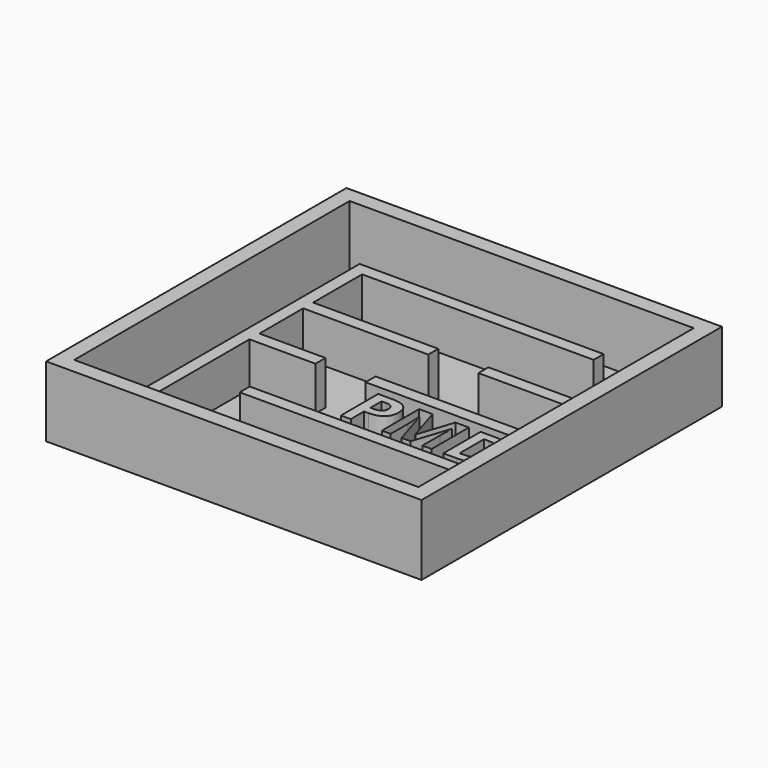
from build123d import *

# Parameters (mm, degrees)
F0_W         = 38.1
F0_H         = 38.1
F1_DEPTH     = 0.79375
F2_W         = 38.1
F2_H         = 38.1
F2_W_2       = 34.925
F2_H_2       = 34.925
F3_DEPTH     = 6.35
F4_R         = 1.27
F5_DEPTH     = 0.396875
F4_W         = 10.795
F4_H         = 1.27
F4_W_2       = 16.7933495293
F4_W_3       = 23.495
F4_W_4       = 12.2181028306
F4_W_5       = 11.1757950872
F6_DEPTH     = 4.445
F4_TEXT_SIZE = 6.6178126468
F7_DEPTH     = 4.445


# Not quite as in the source:
# - Text() gives the source's letters only with a copy of the font that has no kerning and outlines rounded to 1/6400 em; it was checked with that copy


with BuildPart() as f1:
    # F0 (on Top) → F1 (new body)
    with BuildSketch(Plane.XY):
        with Locations((7.1995537728, -11.629379993)):
            Rectangle(F0_W, F0_H)
    extrude(amount=F1_DEPTH)

    # F2 (on face) → F3 (join)
    with BuildSketch(Plane.XY.offset(0.79375)):
        with Locations((7.1995537728, -11.629379993)):
            Rectangle(F2_W, F2_H)
        with Locations((7.1995537728, -11.629379993)):
            Rectangle(F2_W_2, F2_H_2, mode=Mode.SUBTRACT)
    extrude(amount=F3_DEPTH)

    # F4 (on face) → F5 (cut)
    with BuildSketch(Plane.XY.offset(0.79375)):
        with Locations((-7.7175865881, -26.8155727535)):
            Circle(F4_R)
        with Locations((21.5233564377, -24.9188905582)):
            Circle(F4_R)
    extrude(amount=-F5_DEPTH, mode=Mode.SUBTRACT)

    # F4 (on face) → F6 (join)
    with BuildSketch(Plane.XY.offset(0.79375)):
        Polygon((-5.1829462272, 0.753120007), (-5.1829462272, -29.091879993), (-3.9129462272, -29.091879993), (-3.9129462272, -28.7239273232), (-3.9129462272, -27.4539273232), (-3.9129462272, -14.804379993), (2.7887042435, -14.804379993), (2.7887042435, -13.534379993), (-3.9129462272, -13.534379993), (-3.9129462272, -7.992786257), (8.7870537728, -7.992786257), (8.7870537728, -6.722786257), (-3.9129462272, -6.722786257), (-3.9129462272, -0.516879993), (19.5820537728, -0.516879993), (19.5820537728, 0.753120007), align=None)
        with Locations((19.2645537728, -7.357786257)):
            Rectangle(F4_W, F4_H)
        with Locations((16.2653790082, -14.169379993)):
            Rectangle(F4_W_2, F4_H)
        with Locations((12.9145537728, -21.7488537931)):
            Rectangle(F4_W_3, F4_H)
        with Locations((2.1961051881, -28.0889273232)):
            Rectangle(F4_W_4, F4_H)
        with Locations((19.0741562292, -28.0889273232)):
            Rectangle(F4_W_5, F4_H)
    extrude(amount=F6_DEPTH)

    # F4 (on face) → F7 (join)
    with BuildSketch(Plane.XY.offset(0.79375)):
        with Locations((9.31231305, -20.4796261363)):
            Text('PMD', F4_TEXT_SIZE, font='Open Sans', font_style=FontStyle.BOLD, text_align=(TextAlign.LEFT, TextAlign.BOTTOM))
    extrude(amount=F7_DEPTH)


solid = f1.part
